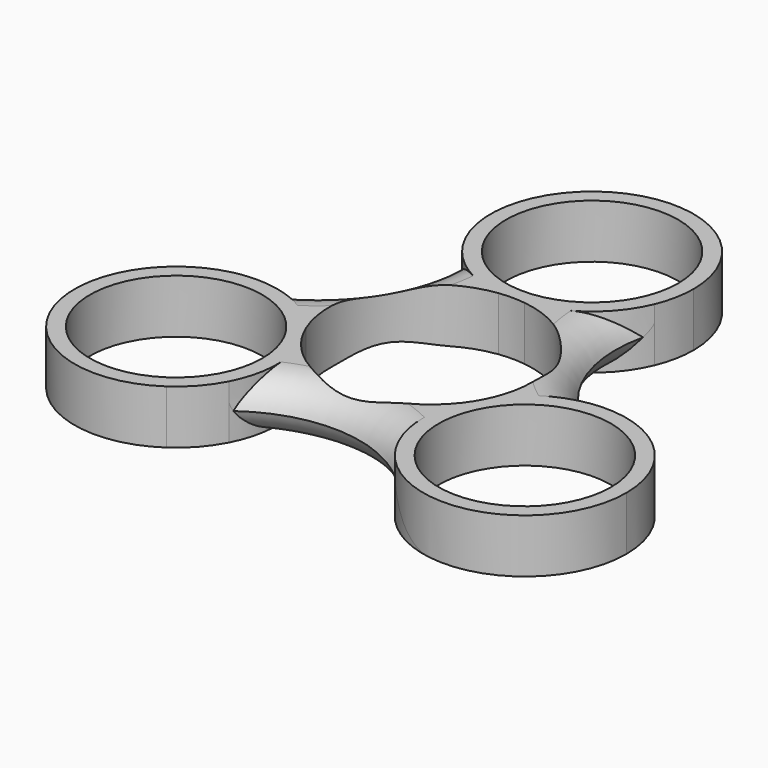
from build123d import *

# Parameters (mm, degrees)
F0_R         = 11.2
F1_DEPTH     = 7
F2_T4_ANGLE  = 168.4949096509
F2_S5_R      = 13.2
F2_T6_DEPTH  = 34
F2_S7_R      = 13.2
F2_T8_DEPTH  = 34
F2_T12_ANGLE = 168.4949096509
F2_S13_R     = 13.2
F2_T14_DEPTH = 34
F2_S15_R     = 13.2
F2_T16_DEPTH = 34
F2_T20_ANGLE = 168.4949096509
F2_S21_R     = 13.2
F2_T22_DEPTH = 28
F2_S23_R     = 13.2
F2_T24_DEPTH = 28
F2_T28_ANGLE = 168.4949096509
F2_S29_R     = 13.2
F2_T30_DEPTH = 28
F2_S31_R     = 13.2
F2_T32_DEPTH = 28
F2_T36_ANGLE = 168.4949096509
F2_S37_R     = 13.2
F2_T38_DEPTH = 28
F2_S39_R     = 13.2
F2_T40_DEPTH = 28
F2_T44_ANGLE = 168.4949096509
F2_S45_R     = 13.2
F2_T46_DEPTH = 28
F2_S47_R     = 13.2
F2_T48_DEPTH = 28


# Not quite as in the source:
# - a fillet or chamfer that OpenCascade refuses, or shapes differently, is made with other operations: its cross-section is extruded or revolved along the edge and cut away or added


with BuildPart() as f1:
    # F0 (on Top) → F1 (new body)
    with BuildSketch(Plane.XY):
        with BuildLine():
            ThreePointArc((1.7091213093, 13.0888847634), (9.9196875274, 8.7086049031), (13.2, 0))
            ThreePointArc((13.2, 0), (12.9450038479, -2.5820293139), (12.189867367, -5.0642999097))
            ThreePointArc((12.189867367, -5.0642999097), (16.5628624938, -1.3869456691), (22.080220354, 0.0979054458))
            ThreePointArc((22.080220354, 0.0979054458), (13.0447596571, 8.6807163883), (12.189867367, 21.1134696171))
            ThreePointArc((12.189867367, 21.1134696171), (8.0245848537, 15.6970234692), (1.7091213093, 13.0888847634))
        make_face()
        with BuildLine():
            ThreePointArc((-1.7091213093, 13.0888847634), (0, 13.2), (1.7091213093, 13.0888847634))
            ThreePointArc((1.7091213093, 13.0888847634), (8.0245848537, 15.6970234692), (12.189867367, 21.1134696171))
            ThreePointArc((12.189867367, 21.1134696171), (12.9450038479, 23.5957402129), (13.2, 26.1777695268))
            ThreePointArc((13.2, 26.1777695268), (-0.5113068084, 39.3678629817), (-13.160388689, 25.1559233773))
            ThreePointArc((-13.160388689, 25.1559233773), (-11.8561925419, 22.2103557846), (-11.1248987802, 19.0730790248))
            ThreePointArc((-11.1248987802, 19.0730790248), (-7.0803010638, 15.0373325136), (-1.7091213093, 13.0888847634))
        make_face()
        with Locations((0, 26.1777695268)):
            Circle(F0_R, mode=Mode.SUBTRACT)
        with BuildLine():
            ThreePointArc((22.080220354, 0.0979054458), (16.5628624938, -1.3869456691), (12.189867367, -5.0642999097))
            ThreePointArc((12.189867367, -5.0642999097), (11.43153533, -6.6), (10.4807460577, -8.0245848537))
            ThreePointArc((10.4807460577, -8.0245848537), (9.5817286612, -14.7980060727), (12.189867367, -21.1134696171))
            ThreePointArc((12.189867367, -21.1134696171), (26.9070123694, -25.5906016047), (35.8706134247, -13.0888847634))
            ThreePointArc((35.8706134247, -13.0888847634), (33.8379160306, -6.0510333508), (28.3658630449, -1.1807307602))
            ThreePointArc((28.3658630449, -1.1807307602), (25.1628286075, -0.8374139589), (22.080220354, 0.0979054458))
        make_face()
        with Locations((22.6706134247, -13.0888847634)):
            Circle(F0_R, mode=Mode.SUBTRACT)
        with BuildLine():
            ThreePointArc((-12.189867367, -5.0642999097), (-11.43153533, 6.6), (-1.7091213093, 13.0888847634))
            ThreePointArc((-1.7091213093, 13.0888847634), (-7.0803010638, 15.0373325136), (-11.1248987802, 19.0730790248))
            ThreePointArc((-11.1248987802, 19.0730790248), (-14.0401007438, 6.9567350552), (-24.379734734, 0))
            ThreePointArc((-24.379734734, 0), (-17.606313515, -0.8990173964), (-12.189867367, -5.0642999097))
        make_face()
        with BuildLine():
            ThreePointArc((12.189867367, -21.1134696171), (9.5817286612, -14.7980060727), (10.4807460577, -8.0245848537))
            ThreePointArc((10.4807460577, -8.0245848537), (0, -13.2), (-10.4807460577, -8.0245848537))
            ThreePointArc((-10.4807460577, -8.0245848537), (-9.7256095768, -10.5068554495), (-9.4706134247, -13.0888847634))
            ThreePointArc((-9.4706134247, -13.0888847634), (-9.8471612289, -16.219231994), (-10.9553215737, -19.1709844706))
            ThreePointArc((-10.9553215737, -19.1709844706), (0.9953410867, -15.6374514435), (12.189867367, -21.1134696171))
        make_face()
        with BuildLine():
            ThreePointArc((28.3658630449, -1.1807307602), (25.3018902506, -0.153801375), (22.080220354, 0.0979054458))
            ThreePointArc((22.080220354, 0.0979054458), (25.1628286075, -0.8374139589), (28.3658630449, -1.1807307602))
        make_face()
        with BuildLine():
            ThreePointArc((-10.4807460577, -8.0245848537), (-11.43153533, -6.6), (-12.189867367, -5.0642999097))
            ThreePointArc((-12.189867367, -5.0642999097), (-17.606313515, -0.8990173964), (-24.379734734, 0))
            ThreePointArc((-24.379734734, 0), (-34.9988493231, -17.8063628643), (-15.2054743558, -23.975192617))
            ThreePointArc((-15.2054743558, -23.975192617), (-13.3066360656, -21.3729418257), (-10.9553215737, -19.1709844706))
            ThreePointArc((-10.9553215737, -19.1709844706), (-9.8471612289, -16.219231994), (-9.4706134247, -13.0888847634))
            ThreePointArc((-9.4706134247, -13.0888847634), (-9.7256095768, -10.5068554495), (-10.4807460577, -8.0245848537))
        make_face()
        with Locations((-22.6706134247, -13.0888847634)):
            Circle(F0_R, mode=Mode.SUBTRACT)
        with BuildLine():
            ThreePointArc((-13.160388689, 25.1559233773), (-12.5177492274, 21.9889804083), (-11.1248987802, 19.0730790248))
            ThreePointArc((-11.1248987802, 19.0730790248), (-11.8561925419, 22.2103557846), (-13.160388689, 25.1559233773))
        make_face()
        with BuildLine():
            ThreePointArc((-15.2054743558, -23.975192617), (-12.7841410232, -21.8351790333), (-10.9553215737, -19.1709844706))
            ThreePointArc((-10.9553215737, -19.1709844706), (-13.3066360656, -21.3729418257), (-15.2054743558, -23.975192617))
        make_face()
    extrude(amount=F1_DEPTH)

    # F2: fillet of radius 5 on 6 edges, made by hand


with BuildPart() as f2_tool2:
    # F2_s3 → F2_t4 (revolve)
    with BuildSketch(Plane(origin=(-24.5289306656, 20.9866691127, 0), x_dir=(0, 0, 1), z_dir=(-0.7598399097, 0.6501102303, 0))):
        with BuildLine():
            ThreePointArc((2, 11.6140074633), (5.5355339059, 13.0784735574), (7, 16.6140074633))
            Line((7, 16.6140074633), (7, 11.6140074633))
            Line((7, 11.6140074633), (2, 11.6140074633))
        make_face()
    revolve(axis=Axis((-28.1457095267, 16.7594276462, 7), (0, 0, -1)), revolution_arc=F2_T4_ANGLE)

    # F2_s5 → F2_t6 (cut, symmetric)
    with BuildSketch(Plane.XY.offset(2.7)):
        with Locations((0, 26.1777695268)):
            Circle(F2_S5_R)
    extrude(amount=F2_T6_DEPTH, both=True, mode=Mode.SUBTRACT)

    # F2_s7 → F2_t8 (cut, symmetric)
    with BuildSketch(Plane.XY.offset(2.7)):
        with Locations((-22.6706134247, -13.0888847634)):
            Circle(F2_S7_R)
    extrude(amount=F2_T8_DEPTH, both=True, mode=Mode.SUBTRACT)


with BuildPart() as f1_1:
    add(f1.part)

    # F2_t1: cut F2_tool2
    add(f2_tool2.part, mode=Mode.SUBTRACT)


with BuildPart() as f2_tool10:
    # F2_s11 → F2_t12 (revolve)
    with BuildSketch(Plane(origin=(-24.5289306656, 20.9866691127, 0), x_dir=(0, 0, 1), z_dir=(-0.7598399097, 0.6501102303, 0))):
        with BuildLine():
            ThreePointArc((5, 11.6140074633), (1.4644660941, 13.0784735574), (0, 16.6140074633))
            Line((0, 16.6140074633), (0, 11.6140074633))
            Line((0, 11.6140074633), (5, 11.6140074633))
        make_face()
    revolve(axis=Axis((-28.1457095267, 16.7594276462, 0), (0, 0, -1)), revolution_arc=F2_T12_ANGLE)

    # F2_s13 → F2_t14 (cut, symmetric)
    with BuildSketch(Plane.XY.offset(4.3)):
        with Locations((0, 26.1777695268)):
            Circle(F2_S13_R)
    extrude(amount=F2_T14_DEPTH, both=True, mode=Mode.SUBTRACT)

    # F2_s15 → F2_t16 (cut, symmetric)
    with BuildSketch(Plane.XY.offset(4.3)):
        with Locations((-22.6706134247, -13.0888847634)):
            Circle(F2_S15_R)
    extrude(amount=F2_T16_DEPTH, both=True, mode=Mode.SUBTRACT)


with BuildPart() as f1_2:
    add(f1_1.part)

    # F2_t9: cut F2_tool10
    add(f2_tool10.part, mode=Mode.SUBTRACT)


with BuildPart() as f2_tool18:
    # F2_s19 → F2_t20 (revolve)
    with BuildSketch(Plane(origin=(-5.9105232596, -31.7360116404, 0), x_dir=(0, 0, 1), z_dir=(-0.1830920198, -0.9830957798, 0))):
        with BuildLine():
            ThreePointArc((5, 11.6140074633), (1.4644660941, 13.0784735574), (0, 16.6140074633))
            Line((0, 16.6140074633), (0, 11.6140074633))
            Line((0, 11.6140074633), (5, 11.6140074633))
        make_face()
    revolve(axis=Axis((-0.4412353312, -32.7546132808, 0), (0, 0, -1)), revolution_arc=F2_T20_ANGLE)

    # F2_s21 → F2_t22 (cut, symmetric)
    with BuildSketch(Plane.XY.offset(4.3)):
        with Locations((-22.6706134247, -13.0888847634)):
            Circle(F2_S21_R)
    extrude(amount=F2_T22_DEPTH, both=True, mode=Mode.SUBTRACT)

    # F2_s23 → F2_t24 (cut, symmetric)
    with BuildSketch(Plane.XY.offset(4.3)):
        with Locations((22.6706134247, -13.0888847634)):
            Circle(F2_S23_R)
    extrude(amount=F2_T24_DEPTH, both=True, mode=Mode.SUBTRACT)


with BuildPart() as f1_3:
    add(f1_2.part)

    # F2_t17: cut F2_tool18
    add(f2_tool18.part, mode=Mode.SUBTRACT)


with BuildPart() as f2_tool26:
    # F2_s27 → F2_t28 (revolve)
    with BuildSketch(Plane(origin=(30.4394539252, 10.7493425277, 0), x_dir=(0, 0, 1), z_dir=(0.9429319296, 0.3329855495, 0))):
        with BuildLine():
            ThreePointArc((5, 11.6140074633), (1.4644660941, 13.0784735574), (0, 16.6140074633))
            Line((0, 16.6140074633), (0, 11.6140074633))
            Line((0, 11.6140074633), (5, 11.6140074633))
        make_face()
    revolve(axis=Axis((28.5869448579, 15.9951856345, 0), (0, 0, -1)), revolution_arc=F2_T28_ANGLE)

    # F2_s29 → F2_t30 (cut, symmetric)
    with BuildSketch(Plane.XY.offset(2.5)):
        with Locations((0, 26.1777695268)):
            Circle(F2_S29_R)
    extrude(amount=F2_T30_DEPTH, both=True, mode=Mode.SUBTRACT)

    # F2_s31 → F2_t32 (cut, symmetric)
    with BuildSketch(Plane.XY.offset(2.5)):
        with Locations((22.6706134247, -13.0888847634)):
            Circle(F2_S31_R)
    extrude(amount=F2_T32_DEPTH, both=True, mode=Mode.SUBTRACT)


with BuildPart() as f1_4:
    add(f1_3.part)

    # F2_t25: cut F2_tool26
    add(f2_tool26.part, mode=Mode.SUBTRACT)


with BuildPart() as f2_tool34:
    # F2_s35 → F2_t36 (revolve)
    with BuildSketch(Plane(origin=(30.4394539252, 10.7493425277, 0), x_dir=(0, 0, 1), z_dir=(0.9429319296, 0.3329855495, 0))):
        with BuildLine():
            ThreePointArc((2, 11.6140074633), (5.5355339059, 13.0784735574), (7, 16.6140074633))
            Line((7, 16.6140074633), (7, 11.6140074633))
            Line((7, 11.6140074633), (2, 11.6140074633))
        make_face()
    revolve(axis=Axis((28.5869448579, 15.9951856345, 7), (0, 0, -1)), revolution_arc=F2_T36_ANGLE)

    # F2_s37 → F2_t38 (cut, symmetric)
    with BuildSketch(Plane.XY.offset(4.5)):
        with Locations((0, 26.1777695268)):
            Circle(F2_S37_R)
    extrude(amount=F2_T38_DEPTH, both=True, mode=Mode.SUBTRACT)

    # F2_s39 → F2_t40 (cut, symmetric)
    with BuildSketch(Plane.XY.offset(4.5)):
        with Locations((22.6706134247, -13.0888847634)):
            Circle(F2_S39_R)
    extrude(amount=F2_T40_DEPTH, both=True, mode=Mode.SUBTRACT)


with BuildPart() as f1_5:
    add(f1_4.part)

    # F2_t33: cut F2_tool34
    add(f2_tool34.part, mode=Mode.SUBTRACT)


with BuildPart() as f2_tool42:
    # F2_s43 → F2_t44 (revolve)
    with BuildSketch(Plane(origin=(-5.9105232596, -31.7360116404, 0), x_dir=(0, 0, 1), z_dir=(-0.1830920198, -0.9830957798, 0))):
        with BuildLine():
            ThreePointArc((2, 11.6140074633), (5.5355339059, 13.0784735574), (7, 16.6140074633))
            Line((7, 16.6140074633), (7, 11.6140074633))
            Line((7, 11.6140074633), (2, 11.6140074633))
        make_face()
    revolve(axis=Axis((-0.4412353312, -32.7546132808, 7), (0, 0, -1)), revolution_arc=F2_T44_ANGLE)

    # F2_s45 → F2_t46 (cut, symmetric)
    with BuildSketch(Plane.XY.offset(2.7)):
        with Locations((-22.6706134247, -13.0888847634)):
            Circle(F2_S45_R)
    extrude(amount=F2_T46_DEPTH, both=True, mode=Mode.SUBTRACT)

    # F2_s47 → F2_t48 (cut, symmetric)
    with BuildSketch(Plane.XY.offset(2.7)):
        with Locations((22.6706134247, -13.0888847634)):
            Circle(F2_S47_R)
    extrude(amount=F2_T48_DEPTH, both=True, mode=Mode.SUBTRACT)


with BuildPart() as f1_6:
    add(f1_5.part)

    # F2_t41: cut F2_tool42
    add(f2_tool42.part, mode=Mode.SUBTRACT)


solid = f1_6.part
